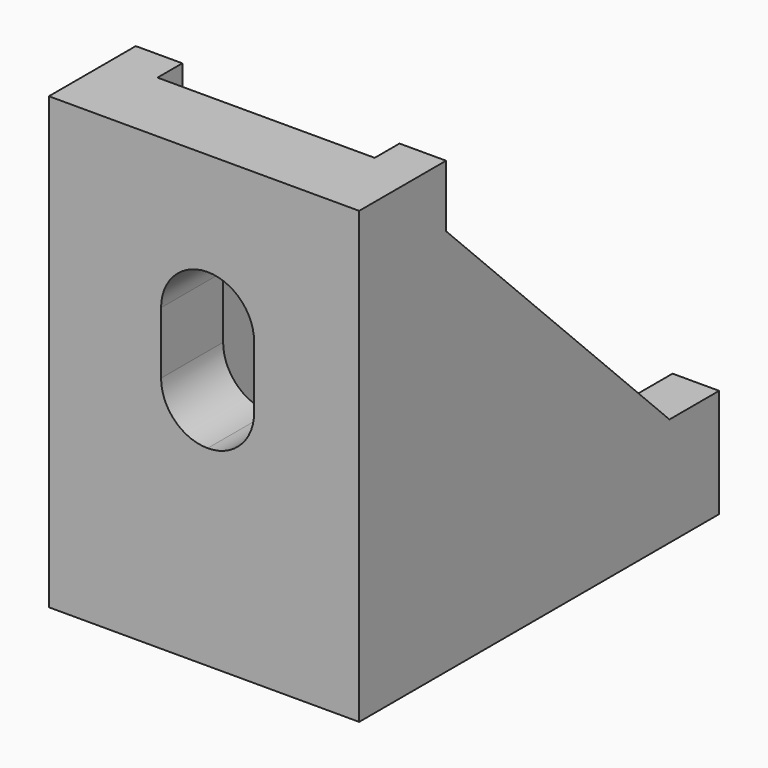
from build123d import *

# Parameters (mm, degrees)
F0_W      = 20
F0_H      = 29
F1_DEPTH  = 5
F3_W      = 20
F3_H      = 24
F4_DEPTH  = 5
F6_DEPTH  = 3
F8_DEPTH  = 3
F9_W      = 6
F9_H      = 10
F10_DEPTH = 29.001
F11_W     = 6
F11_H     = 10
F12_DEPTH = 29.001
F13_R     = 2.99999


# Not quite as in the source:
# - a fillet or chamfer is up to 0.001 mm smaller than in the source, because OpenCascade refuses the exact size


with BuildPart() as f1:
    # F0 (on Top) → F1 (new body)
    with BuildSketch(Plane.XY):
        with Locations((10, 14.5)):
            Rectangle(F0_W, F0_H)
    extrude(amount=F1_DEPTH)

    # F3 (on face) → F4 (join)
    with BuildSketch(Plane.XZ):
        with Locations((10, 17)):
            Rectangle(F3_W, F3_H)
    extrude(amount=-F4_DEPTH)

    # F5 (on face) → F6 (join)
    with BuildSketch(Plane.YZ.offset(20)):
        Polygon((7, 29), (5, 29), (5, 5), (29, 5), (29, 7), (25, 7), (7, 25), align=None)
    extrude(amount=-F6_DEPTH)

    # F7 (on face) → F8 (join)
    with BuildSketch(Plane(origin=(0, 0, 0), x_dir=(0, -1, 0), z_dir=(-1, 0, 0))):
        Polygon((-29, 7), (-29, 5), (-5, 5), (-5, 29), (-7, 29), (-7, 25), (-25, 7), align=None)
    extrude(amount=-F8_DEPTH)

    # F9 (on face) → F10 (cut, through all)
    with BuildSketch(Plane(origin=(0, 0, 0), x_dir=(1, 0, 0), z_dir=(0, 0, -1))):
        with Locations((10, -16)):
            Rectangle(F9_W, F9_H)
    extrude(amount=-F10_DEPTH, mode=Mode.SUBTRACT)

    # F11 (on face) → F12 (cut, through all)
    with BuildSketch(Plane.XZ):
        with Locations((10.2312741801, 17.3546597362)):
            Rectangle(F11_W, F11_H)
    extrude(amount=-F12_DEPTH, mode=Mode.SUBTRACT)

    # F13 (radius 3 in the source; OpenCascade refuses exactly that, so slightly less here)
    f13_edges = [f1.edges().sort_by_distance(p)[0] for p in [
        (7, 11, 2.5),
        (13, 11, 2.5),
        (7, 21, 2.5),
        (13, 21, 2.5),
        (7.231274, 2.5, 12.35466),
        (13.231274, 2.5, 12.35466),
        (7.231274, 2.5, 22.35466),
        (13.231274, 2.5, 22.35466),
    ]]
    fillet(f13_edges, radius=F13_R)


solid = f1.part
